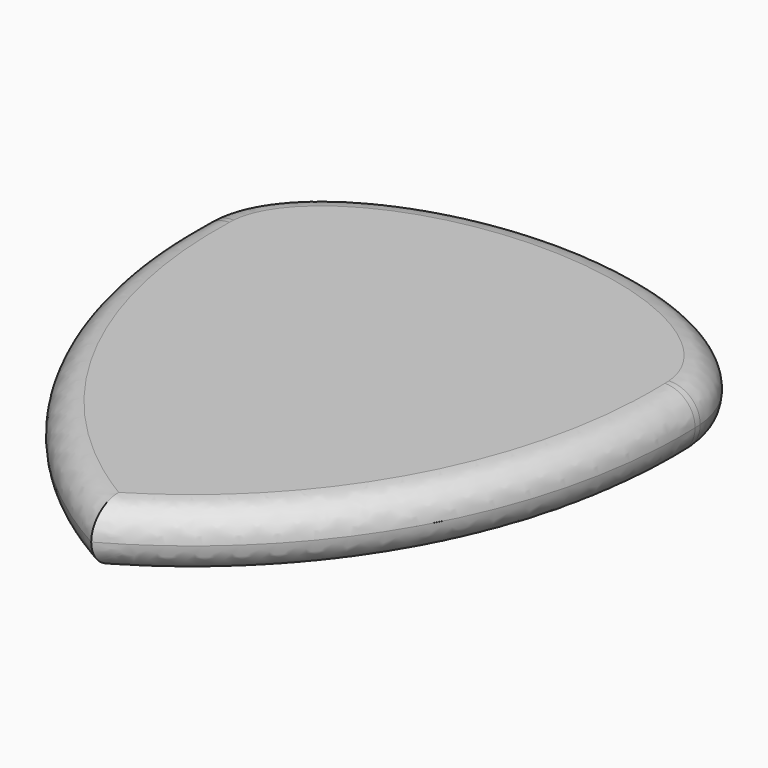
from build123d import *

# Parameters (mm, degrees)
F1_DEPTH = 2.4
F2_R     = 1.1999


# Not quite as in the source:
# - a fillet or chamfer is up to 0.001 mm smaller than in the source, because OpenCascade refuses the exact size


with BuildPart() as f1:
    # F0 (on Top) → F1 (new body)
    with BuildSketch(Plane.XY):
        with BuildLine():
            add(Edge.make_bspline(
                [(-21.6115170717, 0), (-21.6158181441, 0.1367741011), (-21.6219144077, 0.2735359227)],
                knots=[1.0795807164, 1.0795807164, 1.0795807164, 1.0929807321, 1.0929807321, 1.0929807321], degree=2, weights=[1, 0.999977555, 1]))
            add(Edge.make_bspline(
                [(-21.6115170717, 0), (-21.6115170717, 0.1368390995), (-21.6219144077, 0.2735359227)],
                knots=[0, 0, 0, 0.0456051273, 0.0456051273, 0.0456051273], degree=2, weights=[1, 0.9997400328, 1]))
        make_face()
        with BuildLine():
            add(Edge.make_bspline(
                [(-31.6115170717, -18), (-21.2269016871, -12.2307692308), (-21.6115170717, 0)],
                knots=[0, 0, 0, 1.0795807164, 1.0795807164, 1.0795807164], degree=2, weights=[1, 0.8578164469, 1]))
            add(Edge.make_bspline(
                [(-21.6115170717, 0), (-21.6158181441, 0.1367741011), (-21.6219144077, 0.2735359227)],
                knots=[1.0795807164, 1.0795807164, 1.0795807164, 1.0929807321, 1.0929807321, 1.0929807321], degree=2, weights=[1, 0.999977555, 1]))
            add(Edge.make_bspline(
                [(-21.6219144077, 0.2735359227), (-22.0574766194, 6), (-31.6115170717, 6), (-41.165557524, 6), (-41.6011197358, 0.2735359227)],
                knots=[0.0456051273, 0.0456051273, 0.0456051273, 1.5707963268, 1.5707963268, 3.0959875263, 3.0959875263, 3.0959875263], degree=2, weights=[1, 0.7230454068, 1, 0.7230454068, 1]))
            add(Edge.make_bspline(
                [(-41.6011197358, 0.2735359227), (-41.6072159994, 0.1367741011), (-41.6115170717, 0)],
                knots=[5.1902045751, 5.1902045751, 5.1902045751, 5.2036045908, 5.2036045908, 5.2036045908], degree=2, weights=[1, 0.999977555, 1]))
            add(Edge.make_bspline(
                [(-41.6115170717, 0), (-41.9961324563, -12.2307692308), (-31.6115170717, -18)],
                knots=[5.2036045908, 5.2036045908, 5.2036045908, 6.2831853072, 6.2831853072, 6.2831853072], degree=2, weights=[1, 0.8578164469, 1]))
        make_face()
        with BuildLine():
            add(Edge.make_bspline(
                [(-41.6011197358, 0.2735359227), (-41.6072159994, 0.1367741011), (-41.6115170717, 0)],
                knots=[5.1902045751, 5.1902045751, 5.1902045751, 5.2036045908, 5.2036045908, 5.2036045908], degree=2, weights=[1, 0.999977555, 1]))
            add(Edge.make_bspline(
                [(-41.6011197358, 0.2735359227), (-41.6115170717, 0.1368390995), (-41.6115170717, 0)],
                knots=[3.0959875263, 3.0959875263, 3.0959875263, 3.1415926536, 3.1415926536, 3.1415926536], degree=2, weights=[1, 0.9997400328, 1]))
        make_face()
    extrude(amount=F1_DEPTH)

    # F2 (radius 1.2 in the source; OpenCascade refuses exactly that, so slightly less here)
    f2_edges = [f1.edges().sort_by_distance(p)[0] for p in [
        (-31.611517, 6, 2.4),
        (-24.081962, -10.413403, 2.4),
        (-39.141072, -10.413403, 2.4),
        (-31.611517, 6, 0),
        (-24.081962, -10.413403, 0),
        (-39.141072, -10.413403, 0),
    ]]
    fillet(f2_edges, radius=F2_R)


solid = f1.part
